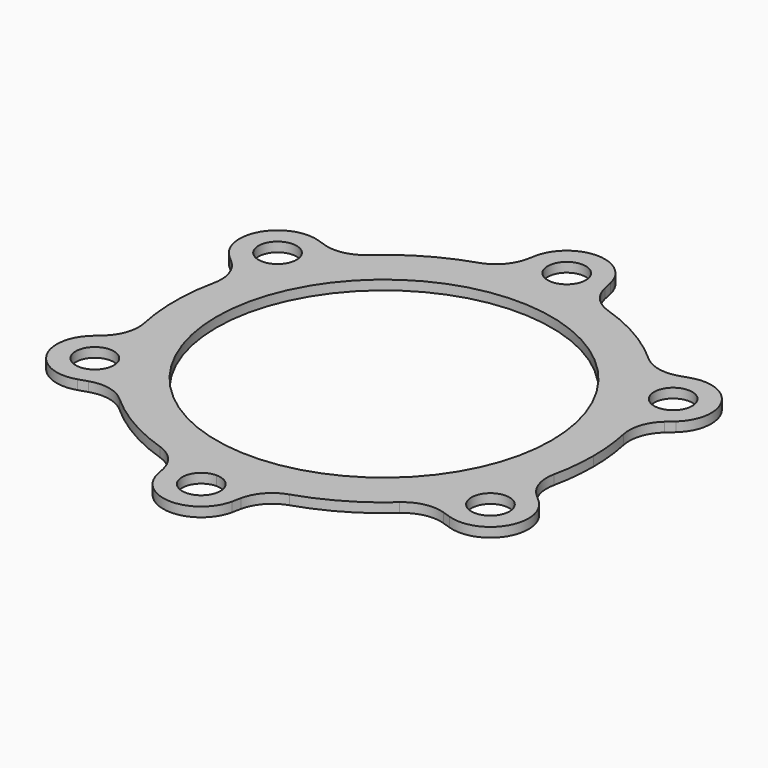
from build123d import *

# Parameters (mm, degrees)
F0_R     = 44
F1_DEPTH = 2.5
F2_R     = 10


# Not quite as in the source:
# - a feature names something its author has since deleted; it is built from what else it names


with BuildPart() as f1:
    # F0 (on Top) → F1 (new body)
    with BuildSketch(Plane.XY):
        with BuildLine():
            ThreePointArc((52.3444859472, -16.8835657052), (54.3320657029, -8.5455623836), (55, 0))
            ThreePointArc((55, 0), (54.3320657029, 8.5455623836), (52.3444859472, 16.8835657052))
            ThreePointArc((52.3444859472, 16.8835657052), (50.268991125, 22.3165528538), (47.6313971166, 27.5000001585))
            ThreePointArc((47.6313971166, 27.5000001585), (44.461197151, 32.3759470579), (40.7938397808, 36.8898717257))
            ThreePointArc((40.7938397808, 36.8898717257), (27.5, 47.6313972081), (11.5506461665, 53.7734374309))
            ThreePointArc((11.5506461665, 53.7734374309), (5.8077939557, 54.6924997542), (-3e-09, 55))
            ThreePointArc((-3e-09, 55), (-5.8077939587, 54.6924997539), (-11.5506461665, 53.7734374309))
            ThreePointArc((-11.5506461665, 53.7734374309), (-27.5, 47.6313972081), (-40.7938397808, 36.8898717257))
            ThreePointArc((-40.7938397808, 36.8898717257), (-44.4611971512, 32.3759470576), (-47.631397117, 27.5000001579))
            ThreePointArc((-47.631397117, 27.5000001579), (-50.2689911251, 22.3165528534), (-52.3444859472, 16.8835657052))
            ThreePointArc((-52.3444859472, 16.8835657052), (-55, 0), (-52.3444859472, -16.8835657052))
            ThreePointArc((-52.3444859472, -16.8835657052), (-50.2689910436, -22.3165530371), (-47.631396916, -27.500000506))
            ThreePointArc((-47.631396916, -27.500000506), (-44.4611970329, -32.3759472201), (-40.7938397808, -36.8898717257))
            ThreePointArc((-40.7938397808, -36.8898717257), (-27.5, -47.6313972081), (-11.5506461665, -53.7734374309))
            ThreePointArc((-11.5506461665, -53.7734374309), (-5.8077939898, -54.6924997506), (-6.55e-08, -55))
            ThreePointArc((-6.55e-08, -55), (5.8077939247, -54.6924997575), (11.5506461665, -53.7734374309))
            ThreePointArc((11.5506461665, -53.7734374309), (27.5, -47.6313972081), (40.7938397808, -36.8898717257))
            ThreePointArc((40.7938397808, -36.8898717257), (44.461197297, -32.3759468575), (47.6313973645, -27.4999997291))
            ThreePointArc((47.6313973645, -27.4999997291), (50.2689912256, -22.3165526272), (52.3444859472, -16.8835657052))
        make_face()
        Circle(F0_R, mode=Mode.SUBTRACT)
        with BuildLine():
            ThreePointArc((-3e-09, 55), (5.8077939557, 54.6924997542), (11.5506461665, 53.7734374309))
            Line((11.5506461665, 53.7734374309), (9.7805788286, 62.0833333333))
            ThreePointArc((9.7805788286, 62.0833333333), (0, 70), (-9.7805788286, 62.0833333333))
            Line((-9.7805788286, 62.0833333333), (-11.5506461665, 53.7734374309))
            ThreePointArc((-11.5506461665, 53.7734374309), (-5.8077939587, 54.6924997539), (-3e-09, 55))
        make_face()
        with BuildLine():
            ThreePointArc((5, 60), (3.5355339049, 56.464466093), (-3e-09, 55))
            ThreePointArc((-3e-09, 55), (-3.5355339049, 63.535533907), (5, 60))
        make_face(mode=Mode.SUBTRACT)
        with BuildLine():
            ThreePointArc((-47.631397117, 27.5000001579), (-44.4611971512, 32.3759470576), (-40.7938397808, 36.8898717257))
            Line((-40.7938397808, 36.8898717257), (-48.875454404, 39.5118963959))
            ThreePointArc((-48.875454404, 39.5118963959), (-60.6217782649, 35), (-58.6560332326, 22.5714369374))
            Line((-58.6560332326, 22.5714369374), (-52.3444859472, 16.8835657052))
            ThreePointArc((-52.3444859472, 16.8835657052), (-50.2689911251, 22.3165528534), (-47.631397117, 27.5000001579))
        make_face()
        with BuildLine():
            ThreePointArc((-46.9615242271, 30), (-47.131895072, 28.7059048625), (-47.631397117, 27.5000001579))
            ThreePointArc((-47.631397117, 27.5000001579), (-56.7911533821, 31.2940951375), (-46.9615242271, 30))
        make_face(mode=Mode.SUBTRACT)
        with BuildLine():
            Line((-48.875454404, -39.5118963959), (-40.7938397808, -36.8898717257))
            ThreePointArc((-40.7938397808, -36.8898717257), (-44.4611970329, -32.3759472201), (-47.631396916, -27.500000506))
            ThreePointArc((-47.631396916, -27.500000506), (-50.2689910436, -22.3165530371), (-52.3444859472, -16.8835657052))
            Line((-52.3444859472, -16.8835657052), (-58.6560332326, -22.5714369374))
            ThreePointArc((-58.6560332326, -22.5714369374), (-60.6217782649, -35), (-48.875454404, -39.5118963959))
        make_face()
        with BuildLine():
            ThreePointArc((-46.9615242271, -30), (-56.7911534341, -31.2940949433), (-47.631396916, -27.500000506))
            ThreePointArc((-47.631396916, -27.500000506), (-47.13189502, -28.7059050567), (-46.9615242271, -30))
        make_face(mode=Mode.SUBTRACT)
        with BuildLine():
            Line((9.7805788286, -62.0833333333), (11.5506461665, -53.7734374309))
            ThreePointArc((11.5506461665, -53.7734374309), (5.8077939247, -54.6924997575), (-6.55e-08, -55))
            ThreePointArc((-6.55e-08, -55), (-5.8077939898, -54.6924997506), (-11.5506461665, -53.7734374309))
            Line((-11.5506461665, -53.7734374309), (-9.7805788286, -62.0833333333))
            ThreePointArc((-9.7805788286, -62.0833333333), (0, -70), (9.7805788286, -62.0833333333))
        make_face()
        with BuildLine():
            ThreePointArc((5, -60), (-3.5355338828, -63.5355339291), (-6.55e-08, -55))
            ThreePointArc((-6.55e-08, -55), (3.5355338828, -56.4644660709), (5, -60))
        make_face(mode=Mode.SUBTRACT)
        with BuildLine():
            Line((58.6560332326, -22.5714369374), (52.3444859472, -16.8835657052))
            ThreePointArc((52.3444859472, -16.8835657052), (50.2689912256, -22.3165526272), (47.6313973645, -27.4999997291))
            ThreePointArc((47.6313973645, -27.4999997291), (44.461197297, -32.3759468575), (40.7938397808, -36.8898717257))
            Line((40.7938397808, -36.8898717257), (48.875454404, -39.5118963959))
            ThreePointArc((48.875454404, -39.5118963959), (60.6217782649, -35), (58.6560332326, -22.5714369374))
        make_face()
        with BuildLine():
            ThreePointArc((56.9615242271, -30), (50.6674288505, -34.829629091), (47.6313973645, -27.4999997291))
            ThreePointArc((47.6313973645, -27.4999997291), (53.2556196037, -25.170370909), (56.9615242271, -30))
        make_face(mode=Mode.SUBTRACT)
        with BuildLine():
            ThreePointArc((47.6313971166, 27.5000001585), (50.268991125, 22.3165528538), (52.3444859472, 16.8835657052))
            Line((52.3444859472, 16.8835657052), (58.6560332326, 22.5714369374))
            ThreePointArc((58.6560332326, 22.5714369374), (60.6217782649, 35), (48.875454404, 39.5118963959))
            Line((48.875454404, 39.5118963959), (40.7938397808, 36.8898717257))
            ThreePointArc((40.7938397808, 36.8898717257), (44.461197151, 32.3759470579), (47.6313971166, 27.5000001585))
        make_face()
        with BuildLine():
            ThreePointArc((56.9615242271, 30), (53.2556193642, 25.1703708449), (47.6313971166, 27.5000001585))
            ThreePointArc((47.6313971166, 27.5000001585), (50.66742909, 34.8296291551), (56.9615242271, 30))
        make_face(mode=Mode.SUBTRACT)
    extrude(amount=F1_DEPTH)

    # F2
    f2_edges = [f1.edges().sort_by_distance(p)[0] for p in [
        (52.344486, -16.883566, 1.25),
        (52.344486, 16.883566, 1.25),
        (40.79384, 36.889872, 1.25),
        (11.550646, 53.773437, 1.25),
        (-11.550646, 53.773437, 1.25),
        (-40.79384, 36.889872, 1.25),
        (-52.344486, 16.883566, 1.25),
        (-52.344486, -16.883566, 1.25),
        (-40.79384, -36.889872, 1.25),
        (-11.550646, -53.773437, 1.25),
        (11.550646, -53.773437, 1.25),
        (40.79384, -36.889872, 1.25),
    ]]
    fillet(f2_edges, radius=F2_R)


solid = f1.part
